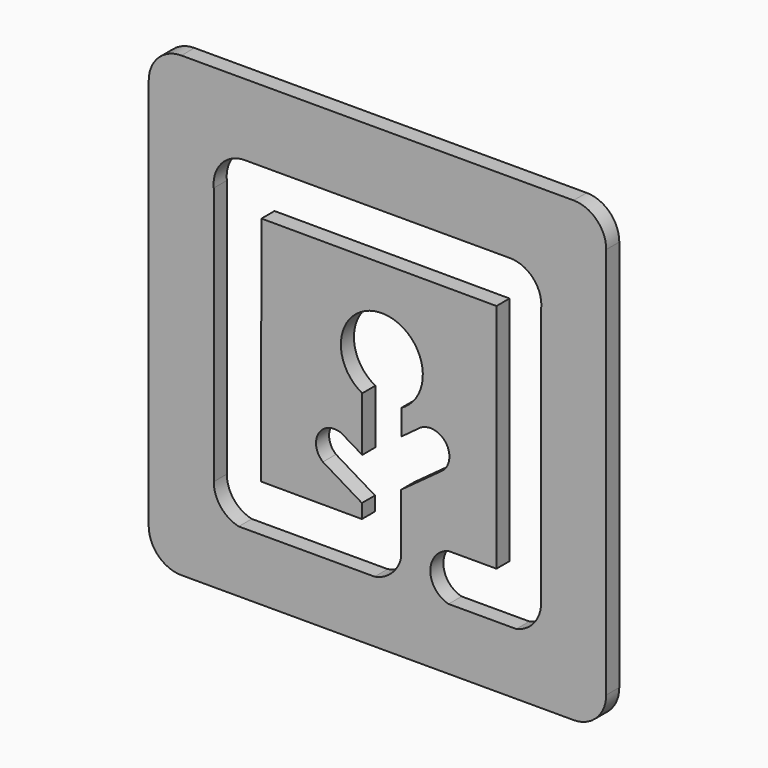
from build123d import *

# Parameters (mm, degrees)
F2_DEPTH = 3.175
F3_DEPTH = 6.35


# Not quite as in the source:
# - a feature of the source that left no trace in its solid (it failed there, or was rolled back) is left out


with BuildPart() as f2:
    # F1 (on Front) → F2 (new body)
    with BuildSketch(Plane.XZ):
        with BuildLine():
            Line((38.1, 38.1), (-38.1, 38.1))
            ThreePointArc((-38.1, 38.1), (-42.5901280605, 36.2401280605), (-44.45, 31.75))
            Line((-44.45, 31.75), (-44.45, -44.45))
            ThreePointArc((-44.45, -44.45), (-42.5901280605, -48.9401280605), (-38.1, -50.8))
            Line((-38.1, -50.8), (38.1, -50.8))
            ThreePointArc((38.1, -50.8), (42.5901280605, -48.9401280605), (44.45, -44.45))
            Line((44.45, -44.45), (44.45, 31.75))
            ThreePointArc((44.45, 31.75), (42.5901280605, 36.2401280605), (38.1, 38.1))
        make_face()
    extrude(amount=F2_DEPTH)

    # F0 (on Front) → F3 (cut)
    with BuildSketch(Plane.XZ):
        with BuildLine():
            Line((-22.538606504, 15.2688146872), (23.1240657176, 15.1560609504))
            Line((23.1240657176, 15.1560609504), (23.1240657176, -29.7829657793))
            Line((23.1240657176, -29.7829657793), (13.8122134028, -29.7829657793))
            ThreePointArc((13.8122134028, -29.7829657793), (10.2694431158, -34.3118906021), (13.8122134028, -38.8408154249))
            Line((13.8122134028, -38.8408154249), (26.9613731652, -38.8408154249))
            ThreePointArc((26.9613731652, -38.8408154249), (30.4505025307, -36.6511380231), (31.8117402494, -32.7632410691))
            Line((31.8117402494, -32.7632410691), (31.8117402494, 17.4764426589))
            ThreePointArc((31.8117402494, 17.4764426589), (30.2845461796, 22.1904359309), (25.758318603, 24.2071952671))
            Line((25.758318603, 24.2071952671), (0, 24.2071952671))
            Line((0, 24.2071952671), (-25.758318603, 24.2071952671))
            ThreePointArc((-25.758318603, 24.2071952671), (-30.2845461796, 22.1904359309), (-31.8117402494, 17.4764426589))
            Line((-31.8117402494, 17.4764426589), (-31.8117402494, -32.7632410691))
            ThreePointArc((-31.8117402494, -32.7632410691), (-30.4505025307, -36.6511380231), (-26.9613731652, -38.8408154249))
            Line((-26.9613731652, -38.8408154249), (-0.5563573561, -38.8408154249))
            ThreePointArc((-0.5563573561, -38.8408154249), (2.7454534653, -37.1689483611), (4.597785615, -33.964894712))
            Line((4.597785615, -33.964894712), (4.597785615, -22.288704291))
            Line((4.597785615, -22.288704291), (12.7450192465, -16.3317304105))
            ThreePointArc((12.7450192465, -16.3317304105), (13.2165532375, -11.3368660938), (8.2683697798, -10.508316569))
            Line((8.2683697798, -10.508316569), (4.6611472023, -13.1736341055))
            Line((4.6611472023, -13.1736341055), (4.6611472023, -8.2560405135))
            ThreePointArc((4.6611472023, -8.2560405135), (0.8511472023, 6.6980150241), (-2.9588527977, -8.2560405135))
            Line((-2.9588527977, -8.2560405135), (-2.9588527977, -18.8035315381))
            Line((-2.9588527977, -18.8035315381), (-7.0704589598, -16.3561142981))
            ThreePointArc((-7.0704589598, -16.3561142981), (-11.4601778268, -17.9054311979), (-10.6000266969, -22.4803797901))
            Line((-10.6000266969, -22.4803797901), (-3.022214385, -27.0476285368))
            Line((-3.022214385, -27.0476285368), (-3.022214385, -29.7946484487))
            Line((-3.022214385, -29.7946484487), (-22.6497609527, -29.7461826206))
            Line((-22.6497609527, -29.7461826206), (-22.538606504, 15.2688146872))
        make_face()
    extrude(amount=F3_DEPTH, mode=Mode.SUBTRACT)


solid = f2.part
